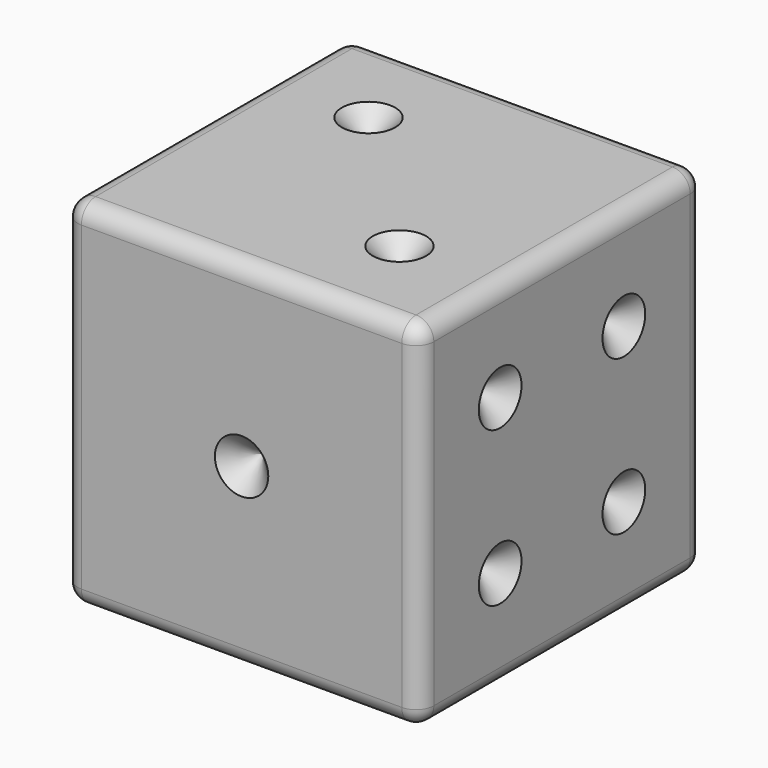
from build123d import *

# Parameters (mm, degrees)
F0_W      = 20
F0_H      = 20
F1_DEPTH  = 20
F2_R      = 1.5
F3_DEPTH  = 1.5
F4_SIZE   = 1.49999
F5_R      = 1.5
F6_DEPTH  = 1.5
F7_SIZE   = 1.49999
F8_SIZE   = 1.49999
F9_R      = 1.5
F10_DEPTH = 1.5
F11_SIZE  = 1.49999
F12_R     = 1.5
F13_DEPTH = 1.5
F14_SIZE  = 1.49999
F15_R     = 1.5
F16_DEPTH = 1.5
F17_SIZE  = 1.49999
F18_R     = 1.5
F19_DEPTH = 1.5
F20_SIZE  = 1.49999
F21_R     = 1


# Not quite as in the source:
# - a fillet or chamfer is up to 0.001 mm smaller than in the source, because OpenCascade refuses the exact size


with BuildPart() as f1:
    # F0 (on Top) → F1 (new body)
    with BuildSketch(Plane.XY):
        with Locations((10, 10)):
            Rectangle(F0_W, F0_H)
    extrude(amount=F1_DEPTH)

    # F2 (on face) → F3 (cut)
    with BuildSketch(Plane.XZ):
        with Locations((10, 10)):
            Circle(F2_R)
    extrude(amount=-F3_DEPTH, mode=Mode.SUBTRACT)

    # F4 (size 1.5 in the source; OpenCascade refuses exactly that, so slightly less here)
    f4_edges = [f1.edges().sort_by_distance(p)[0] for p in [
        (8.5, 1.5, 10),
    ]]
    chamfer(f4_edges, length=F4_SIZE)

    # F5 (on face) → F6 (cut)
    with BuildSketch(Plane.XY.offset(20)):
        with Locations((5.6568542495, 14.3431457505)):
            Circle(F5_R)
        with Locations((14.3431457505, 5.6568542495)):
            Circle(F5_R)
    extrude(amount=-F6_DEPTH, mode=Mode.SUBTRACT)

    # F7 (size 1.5 in the source; OpenCascade refuses exactly that, so slightly less here)
    f7_edges = [f1.edges().sort_by_distance(p)[0] for p in [
        (4.156854, 14.343146, 18.5),
    ]]
    chamfer(f7_edges, length=F7_SIZE)

    # F8 (size 1.5 in the source; OpenCascade refuses exactly that, so slightly less here)
    f8_edges = [f1.edges().sort_by_distance(p)[0] for p in [
        (12.843146, 5.656854, 18.5),
    ]]
    chamfer(f8_edges, length=F8_SIZE)

    # F9 (on face) → F10 (cut)
    with BuildSketch(Plane(origin=(0, 0, 0), x_dir=(0, -1, 0), z_dir=(-1, 0, 0))):
        with Locations((-14.3431457505, 14.3431457505)):
            Circle(F9_R)
        with Locations((-10, 10)):
            Circle(F9_R)
        with Locations((-5.6568542495, 5.6568542495)):
            Circle(F9_R)
    extrude(amount=-F10_DEPTH, mode=Mode.SUBTRACT)

    # F11 (size 1.5 in the source; OpenCascade refuses exactly that, so slightly less here)
    f11_edges = [f1.edges().sort_by_distance(p)[0] for p in [
        (1.5, 15.843146, 14.343146),
        (1.5, 11.5, 10),
        (1.5, 7.156854, 5.656854),
    ]]
    chamfer(f11_edges, length=F11_SIZE)

    # F12 (on face) → F13 (cut)
    with BuildSketch(Plane.YZ.offset(20)):
        with Locations((5.6568542495, 14.3431457505)):
            Circle(F12_R)
        with Locations((14.3431457505, 14.3431457505)):
            Circle(F12_R)
        with Locations((14.3431457505, 5.6568542495)):
            Circle(F12_R)
        with Locations((5.6568542495, 5.6568542495)):
            Circle(F12_R)
    extrude(amount=-F13_DEPTH, mode=Mode.SUBTRACT)

    # F14 (size 1.5 in the source; OpenCascade refuses exactly that, so slightly less here)
    f14_edges = [f1.edges().sort_by_distance(p)[0] for p in [
        (18.5, 4.156854, 14.343146),
        (18.5, 12.843146, 14.343146),
        (18.5, 12.843146, 5.656854),
        (18.5, 4.156854, 5.656854),
    ]]
    chamfer(f14_edges, length=F14_SIZE)

    # F15 (on face) → F16 (cut)
    with BuildSketch(Plane(origin=(0, 0, 0), x_dir=(1, 0, 0), z_dir=(0, 0, -1))):
        with Locations((5.6568542495, -5.6568542495)):
            Circle(F15_R)
        with Locations((10, -10)):
            Circle(F15_R)
        with Locations((14.3431457505, -5.6568542495)):
            Circle(F15_R)
        with Locations((14.3431457505, -14.3431457505)):
            Circle(F15_R)
        with Locations((5.6568542495, -14.3431457505)):
            Circle(F15_R)
    extrude(amount=-F16_DEPTH, mode=Mode.SUBTRACT)

    # F17 (size 1.5 in the source; OpenCascade refuses exactly that, so slightly less here)
    f17_edges = [f1.edges().sort_by_distance(p)[0] for p in [
        (4.156854, 5.656854, 1.5),
        (12.843146, 5.656854, 1.5),
        (8.5, 10, 1.5),
        (4.156854, 14.343146, 1.5),
        (12.843146, 14.343146, 1.5),
    ]]
    chamfer(f17_edges, length=F17_SIZE)

    # F18 (on face) → F19 (cut)
    with BuildSketch(Plane(origin=(0, 20, 0), x_dir=(-1, 0, 0), z_dir=(0, 1, 0))):
        with Locations((-14.3431457505, 14.3431457505)):
            Circle(F18_R)
        with Locations((-5.6568542495, 14.3431457505)):
            Circle(F18_R)
        with Locations((-5.6568542495, 10)):
            Circle(F18_R)
        with Locations((-14.3431457505, 10)):
            Circle(F18_R)
        with Locations((-14.3431457505, 5.6568542495)):
            Circle(F18_R)
        with Locations((-5.6568542495, 5.6568542495)):
            Circle(F18_R)
    extrude(amount=-F19_DEPTH, mode=Mode.SUBTRACT)

    # F20 (size 1.5 in the source; OpenCascade refuses exactly that, so slightly less here)
    f20_edges = [f1.edges().sort_by_distance(p)[0] for p in [
        (15.843146, 18.5, 14.343146),
        (7.156854, 18.5, 14.343146),
        (7.156854, 18.5, 10),
        (15.843146, 18.5, 10),
        (15.843146, 18.5, 5.656854),
        (7.156854, 18.5, 5.656854),
    ]]
    chamfer(f20_edges, length=F20_SIZE)

    # F21
    f21_edges = [f1.edges().sort_by_distance(p)[0] for p in [
        (0, 10, 20),
        (10, 0, 20),
        (20, 10, 20),
        (10, 20, 20),
        (20, 20, 10),
        (20, 0, 10),
        (0, 0, 10),
        (20, 10, 0),
        (10, 0, 0),
        (0, 20, 10),
        (0, 10, 0),
        (10, 20, 0),
    ]]
    fillet(f21_edges, radius=F21_R)


solid = f1.part
